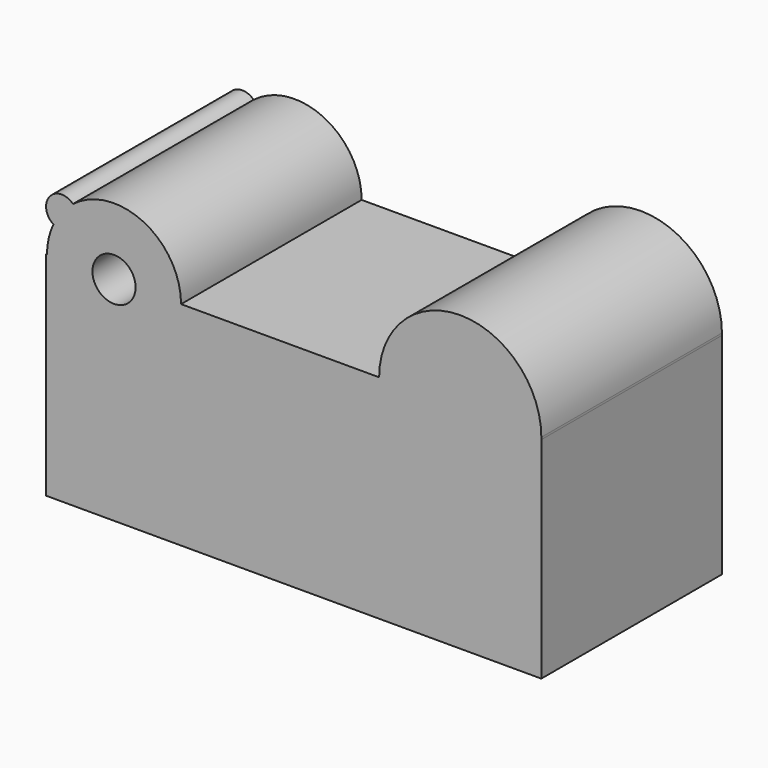
from build123d import *

# Parameters (mm, degrees)
F1_DEPTH = 25.4
F3_DEPTH = 25.4


# Not quite as in the source:
# - the program builds the solid bodies; features that only make, move or delete a surface that nothing else refers to are left out


with BuildPart() as f1:
    # F0 (on Front) → F1 (new body)
    with BuildSketch(Plane.XZ):
        with BuildLine():
            Line((9.6126659133, 12.4514792114), (-12.6748333757, 12.4514792114))
            ThreePointArc((-12.6748333757, 12.4514792114), (-20.2182408326, 4.9080717545), (-27.7616482896, 12.4514792114))
            Line((-27.7616482896, 12.4514792114), (-27.861725539, 12.4514792114))
            Line((-27.861725539, 12.4514792114), (-27.861725539, -11.4652235061))
            Line((-27.861725539, -11.4652235061), (27.8617236763, -11.4652235061))
            Line((27.8617236763, -11.4652235061), (27.8617236763, 12.2047088224))
            ThreePointArc((27.8617236763, 12.2047088224), (18.6154667795, 3.3261161383), (9.6126659133, 12.4514792114))
        make_face()
        with BuildLine():
            Line((-12.6748333757, 12.4514792114), (-17.7898686341, 12.4514792114))
            ThreePointArc((-17.7898686341, 12.4514792114), (-20.2182408326, 10.0231070129), (-22.6466130312, 12.4514792114))
            Line((-22.6466130312, 12.4514792114), (-27.7616482896, 12.4514792114))
            ThreePointArc((-27.7616482896, 12.4514792114), (-20.2182408326, 4.9080717545), (-12.6748333757, 12.4514792114))
        make_face()
    extrude(amount=F1_DEPTH)

    # F0 (on Front) → F3 (join)
    with BuildSketch(Plane.XZ):
        with BuildLine():
            ThreePointArc((-22.6466130312, 12.4514792114), (-20.2182408326, 14.87985141), (-17.7898686341, 12.4514792114))
            Line((-17.7898686341, 12.4514792114), (-12.6748333757, 12.4514792114))
            ThreePointArc((-12.6748333757, 12.4514792114), (-16.8959093658, 19.2238576479), (-24.8351495055, 18.4169758688))
            ThreePointArc((-24.8351495055, 18.4169758688), (-24.460861538, 17.8481513463), (-24.3295943797, 17.1800033439))
            ThreePointArc((-24.3295943797, 17.1800033439), (-25.2407357632, 15.634657994), (-27.0340151871, 15.6838492415))
            ThreePointArc((-27.0340151871, 15.6838492415), (-27.5774921245, 14.1081072584), (-27.7616482896, 12.4514792114))
            Line((-27.7616482896, 12.4514792114), (-22.6466130312, 12.4514792114))
        make_face()
        with BuildLine():
            Line((-12.6748333757, 12.4514792114), (-17.7898686341, 12.4514792114))
            ThreePointArc((-17.7898686341, 12.4514792114), (-20.2182408326, 10.0231070129), (-22.6466130312, 12.4514792114))
            Line((-22.6466130312, 12.4514792114), (-27.7616482896, 12.4514792114))
            ThreePointArc((-27.7616482896, 12.4514792114), (-20.2182408326, 4.9080717545), (-12.6748333757, 12.4514792114))
        make_face()
        with BuildLine():
            Line((9.6126659133, 12.4514792114), (-12.6748333757, 12.4514792114))
            ThreePointArc((-12.6748333757, 12.4514792114), (-20.2182408326, 4.9080717545), (-27.7616482896, 12.4514792114))
            Line((-27.7616482896, 12.4514792114), (-27.861725539, 12.4514792114))
            Line((-27.861725539, 12.4514792114), (-27.861725539, -11.4652235061))
            Line((-27.861725539, -11.4652235061), (27.8617236763, -11.4652235061))
            Line((27.8617236763, -11.4652235061), (27.8617236763, 12.2047088224))
            ThreePointArc((27.8617236763, 12.2047088224), (18.6154667795, 3.3261161383), (9.6126659133, 12.4514792114))
        make_face()
        with BuildLine():
            ThreePointArc((27.8650605952, 12.4514792114), (18.7388632542, 21.5776765524), (9.6126659133, 12.4514792114))
            Line((9.6126659133, 12.4514792114), (27.8617236763, 12.4514792114))
            Line((27.8617236763, 12.4514792114), (27.8617236763, 12.2047088224))
            ThreePointArc((27.8617236763, 12.2047088224), (27.8642263273, 12.3280827367), (27.8650605952, 12.4514792114))
        make_face()
        with BuildLine():
            Line((27.8617236763, 12.4514792114), (9.6126659133, 12.4514792114))
            ThreePointArc((9.6126659133, 12.4514792114), (18.6154667795, 3.3261161383), (27.8617236763, 12.2047088224))
            Line((27.8617236763, 12.2047088224), (27.8617236763, 12.4514792114))
        make_face()
        with BuildLine():
            ThreePointArc((-24.3295943797, 17.1800033439), (-24.460861538, 17.8481513463), (-24.8351495055, 18.4169758688))
            ThreePointArc((-24.8351495055, 18.4169758688), (-26.0956599593, 17.1800033439), (-27.0340151871, 15.6838492415))
            ThreePointArc((-27.0340151871, 15.6838492415), (-25.2407357632, 15.634657994), (-24.3295943797, 17.1800033439))
        make_face()
        with BuildLine():
            ThreePointArc((-27.0340151871, 15.6838492415), (-26.0956599593, 17.1800033439), (-24.8351495055, 18.4169758688))
            ThreePointArc((-24.8351495055, 18.4169758688), (-27.4716836828, 18.2870473105), (-27.0340151871, 15.6838492415))
        make_face()
    extrude(amount=F3_DEPTH)


solid = f1.part
